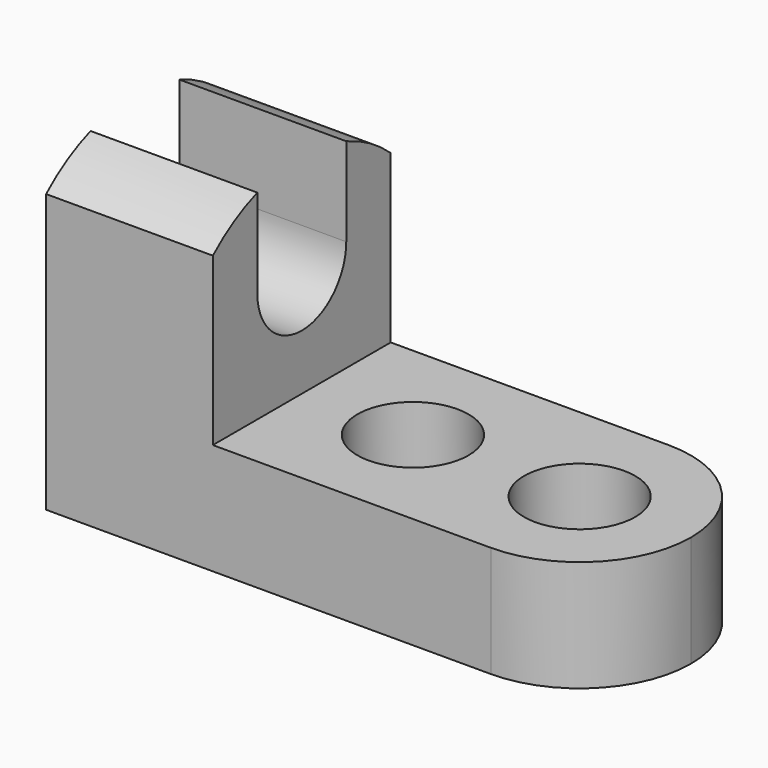
from build123d import *

# Parameters (mm, degrees)
F1_DEPTH  = 25.4
F2_R      = 6.35
F3_DEPTH  = 25.4
F5_DEPTH  = 25.4
F8_DEPTH  = 25.4
F10_DEPTH = 25.4


with BuildPart() as f1:
    # F0 (on Front) → F1 (new body)
    with BuildSketch(Plane.XZ):
        Polygon((0, 38.1), (0, 0), (63.5, 0), (63.5, 12.7), (19.05, 12.7), (19.05, 38.1), align=None)
    extrude(amount=F1_DEPTH)

    # F2 (on face) → F3 (cut)
    with BuildSketch(Plane.XY.offset(12.7)):
        with Locations((31.7500038045, -12.7)):
            Circle(F2_R)
        with Locations((50.8, -12.7120396)):
            Circle(F2_R)
    extrude(amount=-F3_DEPTH, mode=Mode.SUBTRACT)

    # F4 (on face) → F5 (cut)
    with BuildSketch(Plane.XY.offset(12.7)):
        with BuildLine():
            ThreePointArc((63.5, -12.7), (59.7802561211, -21.6802561211), (50.8, -25.4))
            Line((50.8, -25.4), (63.5, -25.4))
            Line((63.5, -25.4), (63.5, -12.7))
        make_face()
        with BuildLine():
            ThreePointArc((50.8, 0), (59.7802561211, -3.7197438789), (63.5, -12.7))
            Line((63.5, -12.7), (63.5, 0))
            Line((63.5, 0), (50.8, 0))
        make_face()
    extrude(amount=-F5_DEPTH, mode=Mode.SUBTRACT)

    # F7 (on face) → F8 (cut)
    with BuildSketch(Plane.YZ.offset(19.05)):
        with BuildLine():
            ThreePointArc((-19.05, 25.4), (-12.7, 19.05), (-6.35, 25.4))
            ThreePointArc((-6.35, 25.4), (-12.7, 31.75), (-19.05, 25.4))
        make_face()
        with BuildLine():
            ThreePointArc((-19.05, 25.4), (-12.7, 31.75), (-6.35, 25.4))
            Line((-6.35, 25.4), (-6.35, 38.1))
            Line((-6.35, 38.1), (-19.05, 38.1))
            Line((-19.05, 38.1), (-19.05, 25.4))
        make_face()
    extrude(amount=-F8_DEPTH, mode=Mode.SUBTRACT)

    # F9 (on face) → F10 (cut)
    with BuildSketch(Plane.YZ.offset(19.05)):
        with BuildLine():
            ThreePointArc((-25.4, 31.75), (-12.7, 36.6009683429), (0, 31.75))
            Line((0, 31.75), (0, 38.1))
            Line((0, 38.1), (-25.4, 38.1))
            Line((-25.4, 38.1), (-25.4, 31.75))
        make_face()
    extrude(amount=-F10_DEPTH, mode=Mode.SUBTRACT)


solid = f1.part
